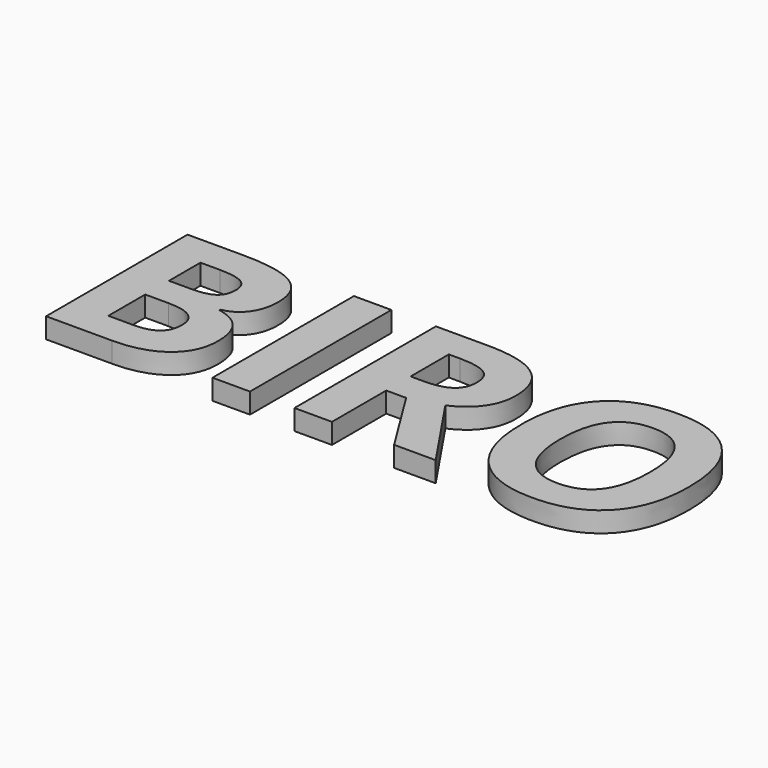
from build123d import *

# Parameters (mm, degrees)
F0_TEXT_SIZE = 24.3330587415
F1_DEPTH     = 2


# Not quite as in the source:
# - Text() gives the source's letters only with a copy of the font that has no kerning and outlines rounded to 1/6400 em; it was checked with that copy


with BuildPart() as f1:
    # F0 (on Top) → F1 (new body)
    with BuildSketch(Plane.XY):
        with Locations((-25.0865161692, -11.7527535487)):
            Text('BIRO', F0_TEXT_SIZE, font='Open Sans', font_style=FontStyle.BOLD, text_align=(TextAlign.LEFT, TextAlign.BOTTOM))
    extrude(amount=F1_DEPTH)


solid = f1.part
